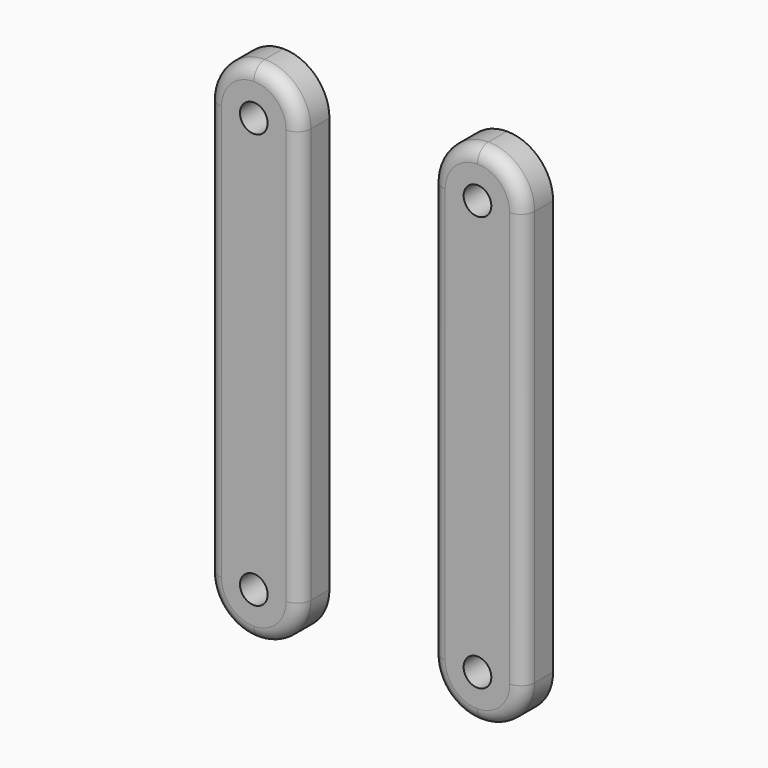
from build123d import *

# Parameters (mm, degrees)
F0_W     = 10
F0_H     = 55
F1_DEPTH = 4
F3_D     = 3
F3_2_D   = 3
F4_R     = 4.99999
F4_2_R   = 4.99999
F5_R     = 1.5
F5_2_R   = 1.5


# Not quite as in the source:
# - a fillet or chamfer is up to 0.001 mm smaller than in the source, because OpenCascade refuses the exact size


with BuildPart() as f1:
    # F0 (on Front) → F1 (new body)
    with BuildSketch(Plane.XZ):
        with Locations((5, 27.5)):
            Rectangle(F0_W, F0_H)
    extrude(amount=F1_DEPTH)

    # F3 (through all)
    with Locations(Plane(origin=(0, 0, 0), x_dir=(1, 0, 0), z_dir=(0, 1, 0))):
        with Locations((5, -50), (29.2528691568, -50), (5, -5), (29.2528691568, -5)):
            Hole(F3_D / 2)

    # F4 (radius 5 in the source; OpenCascade refuses exactly that, so slightly less here)
    f4_edges = [f1.edges().sort_by_distance(p)[0] for p in [
        (0, -2, 55),
        (0, -2, 0),
        (10, -2, 0),
        (10, -2, 55),
    ]]
    fillet(f4_edges, radius=F4_R)

    # F5
    f5_edges = [f1.edges().sort_by_distance(p)[0] for p in [
        (0, -4, 27.5),
    ]]
    fillet(f5_edges, radius=F5_R)


with BuildPart() as f1b:
    # F0 (on Front) → F1, piece 2 (new body)
    with BuildSketch(Plane.XZ):
        with Locations((29.2528691568, 27.5)):
            Rectangle(F0_W, F0_H)
    extrude(amount=F1_DEPTH)

    # F3#2 (through all)
    with Locations(Plane(origin=(0, 0, 0), x_dir=(1, 0, 0), z_dir=(0, 1, 0))):
        with Locations((5, -50), (29.2528691568, -50), (5, -5), (29.2528691568, -5)):
            Hole(F3_2_D / 2)

    # F4#2 (radius 5 in the source; OpenCascade refuses exactly that, so slightly less here)
    f4_2_edges = [f1b.edges().sort_by_distance(p)[0] for p in [
        (24.252869, -2, 55),
        (24.252869, -2, 0),
        (34.252869, -2, 0),
        (34.252869, -2, 55),
    ]]
    fillet(f4_2_edges, radius=F4_2_R)

    # F5#2
    f5_2_edges = [f1b.edges().sort_by_distance(p)[0] for p in [
        (24.252869, -4, 27.5),
    ]]
    fillet(f5_2_edges, radius=F5_2_R)


solid = Compound([f1.part, f1b.part])
